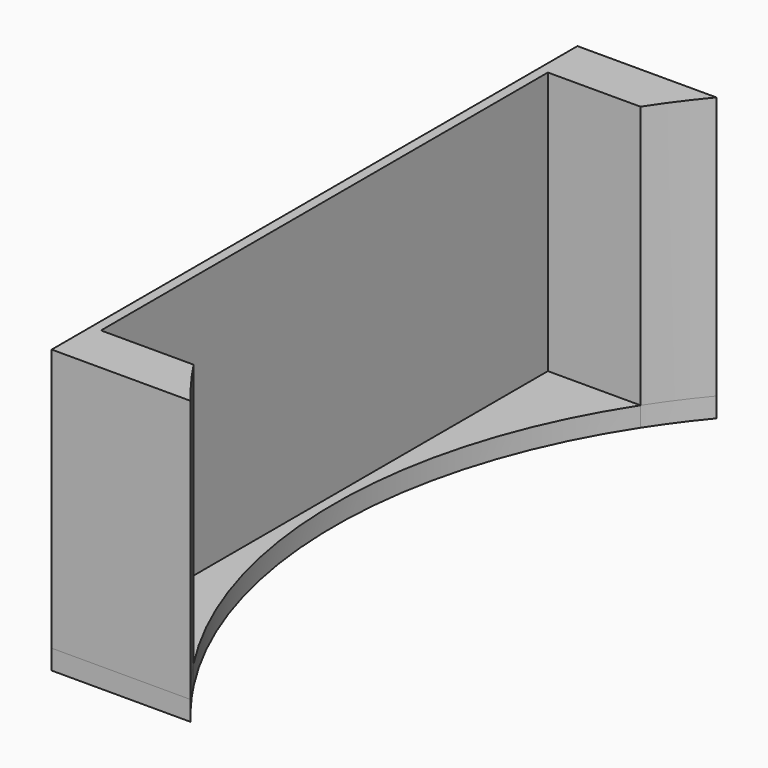
from build123d import *

# Parameters (mm, degrees)
F1_DEPTH = 3
F2_DEPTH = 40


with BuildPart() as f1:
    # F0 (on Top) → F1 (new body)
    with BuildSketch(Plane.XY):
        with BuildLine():
            Line((-126.8924768851, 50.456767044), (-145.0232239954, 50.456767044))
            Line((-145.0232239954, 50.456767044), (-146.5232239827, 50.4565720597))
            Line((-146.5232239827, 50.4565720597), (-146.5232239827, 42.9567671074))
            Line((-146.5232239827, 42.9567671074), (-132.4272471595, 42.958404326))
            ThreePointArc((-132.4272471595, 42.958404326), (-129.7719511525, 46.7903220915), (-126.8924768851, 50.456767044))
        make_face()
        Polygon((-146.5232239827, 42.9567671074), (-146.5232239827, 50.4565720597), (-148.02322397, 50.4563770754), (-148.02322397, -49.5432321111), (-146.5232239827, -49.5432321111), (-146.5232239827, -42.0432321745), align=None)
        with BuildLine():
            Line((-145.0102250409, -49.5432321111), (-126.8755409492, -49.5432321111))
            ThreePointArc((-126.8755409492, -49.5432321111), (-129.7580814774, -45.8752925216), (-132.4161980482, -42.0415949559))
            Line((-132.4161980482, -42.0415949559), (-146.5232239827, -42.0432321745))
            Line((-146.5232239827, -42.0432321745), (-146.5232239827, -49.5432321111))
            Line((-146.5232239827, -49.5432321111), (-145.0102250409, -49.5432321111))
        make_face()
        with BuildLine():
            ThreePointArc((-132.4161980482, -42.0415949559), (-145.0167245182, 0.4567674665), (-132.4272471595, 42.958404326))
            Line((-132.4272471595, 42.958404326), (-146.5232239827, 42.9567671074))
            Line((-146.5232239827, 42.9567671074), (-146.5232239827, -42.0432321745))
            Line((-146.5232239827, -42.0432321745), (-132.4161980482, -42.0415949559))
        make_face()
    extrude(amount=-F1_DEPTH)

    # F0 (on Top) → F2 (join)
    with BuildSketch(Plane.XY):
        with BuildLine():
            Line((-126.8924768851, 50.456767044), (-145.0232239954, 50.456767044))
            Line((-145.0232239954, 50.456767044), (-146.5232239827, 50.4565720597))
            Line((-146.5232239827, 50.4565720597), (-146.5232239827, 42.9567671074))
            Line((-146.5232239827, 42.9567671074), (-132.4272471595, 42.958404326))
            ThreePointArc((-132.4272471595, 42.958404326), (-129.7719511525, 46.7903220915), (-126.8924768851, 50.456767044))
        make_face()
        with BuildLine():
            Line((-145.0102250409, -49.5432321111), (-126.8755409492, -49.5432321111))
            ThreePointArc((-126.8755409492, -49.5432321111), (-129.7580814774, -45.8752925216), (-132.4161980482, -42.0415949559))
            Line((-132.4161980482, -42.0415949559), (-146.5232239827, -42.0432321745))
            Line((-146.5232239827, -42.0432321745), (-146.5232239827, -49.5432321111))
            Line((-146.5232239827, -49.5432321111), (-145.0102250409, -49.5432321111))
        make_face()
        Polygon((-146.5232239827, 42.9567671074), (-146.5232239827, 50.4565720597), (-148.02322397, 50.4563770754), (-148.02322397, -49.5432321111), (-146.5232239827, -49.5432321111), (-146.5232239827, -42.0432321745), align=None)
    extrude(amount=F2_DEPTH)


solid = f1.part
